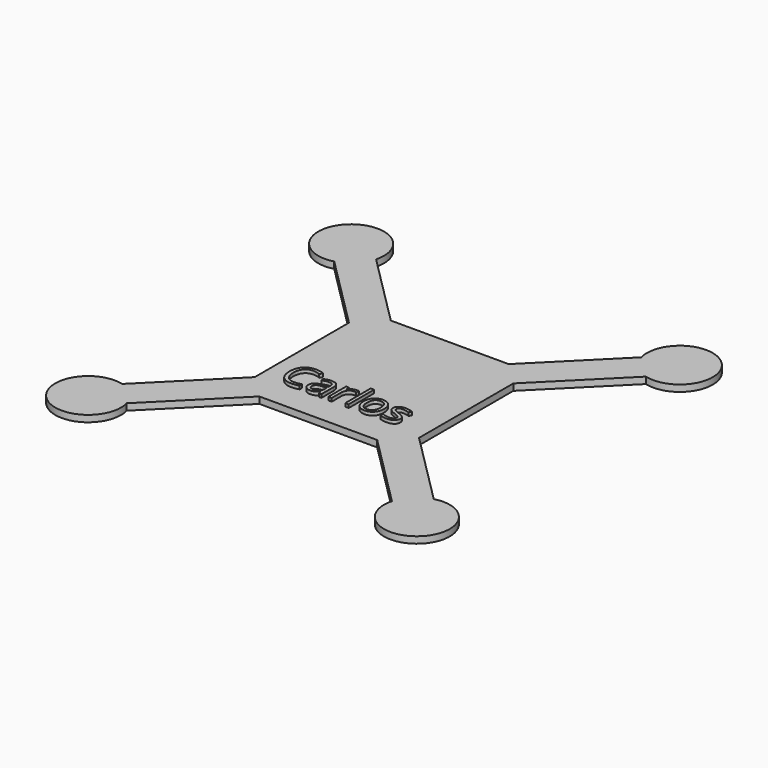
from build123d import *

# Parameters (mm, degrees)
F1_DEPTH     = 2
F2_TEXT_SIZE = 12.6773620852
F3_DEPTH     = 1


# Not quite as in the source:
# - Text() gives the source's letters only with a copy of the font that has no kerning and outlines rounded to 1/6400 em; it was checked with that copy


with BuildPart() as f1:
    # F0 (on Top) → F1 (new body)
    with BuildSketch(Plane.XY):
        with BuildLine():
            Line((-40.3407417371, -47.411809549), (-17.9289321881, -25))
            Line((-17.9289321881, -25), (17.9289321881, -25))
            Line((17.9289321881, -25), (40.3407417371, -47.411809549))
            ThreePointArc((40.3407417371, -47.411809549), (57.0710678119, -57.0710678119), (47.411809549, -40.3407417371))
            Line((47.411809549, -40.3407417371), (25, -17.9289321881))
            Line((25, -17.9289321881), (25, 17.9289321881))
            Line((25, 17.9289321881), (47.411809549, 40.3407417371))
            ThreePointArc((47.411809549, 40.3407417371), (57.0710678119, 57.0710678119), (40.3407417371, 47.411809549))
            Line((40.3407417371, 47.411809549), (17.9289321881, 25))
            Line((17.9289321881, 25), (-17.9289321881, 25))
            Line((-17.9289321881, 25), (-40.3407417371, 47.411809549))
            ThreePointArc((-40.3407417371, 47.411809549), (-57.0710678119, 57.0710678119), (-47.411809549, 40.3407417371))
            Line((-47.411809549, 40.3407417371), (-25, 17.9289321881))
            Line((-25, 17.9289321881), (-25, -17.9289321881))
            Line((-25, -17.9289321881), (-47.411809549, -40.3407417371))
            ThreePointArc((-47.411809549, -40.3407417371), (-57.0710678119, -57.0710678119), (-40.3407417371, -47.411809549))
        make_face()
    extrude(amount=F1_DEPTH)

    # F2 (on face) → F3 (join)
    with BuildSketch(Plane.XY.offset(2)):
        with Locations((-19.9668444693, -16.4013374597)):
            Text('Carlos', F2_TEXT_SIZE, font='Open Sans', text_align=(TextAlign.LEFT, TextAlign.BOTTOM))
    extrude(amount=F3_DEPTH)


solid = f1.part
